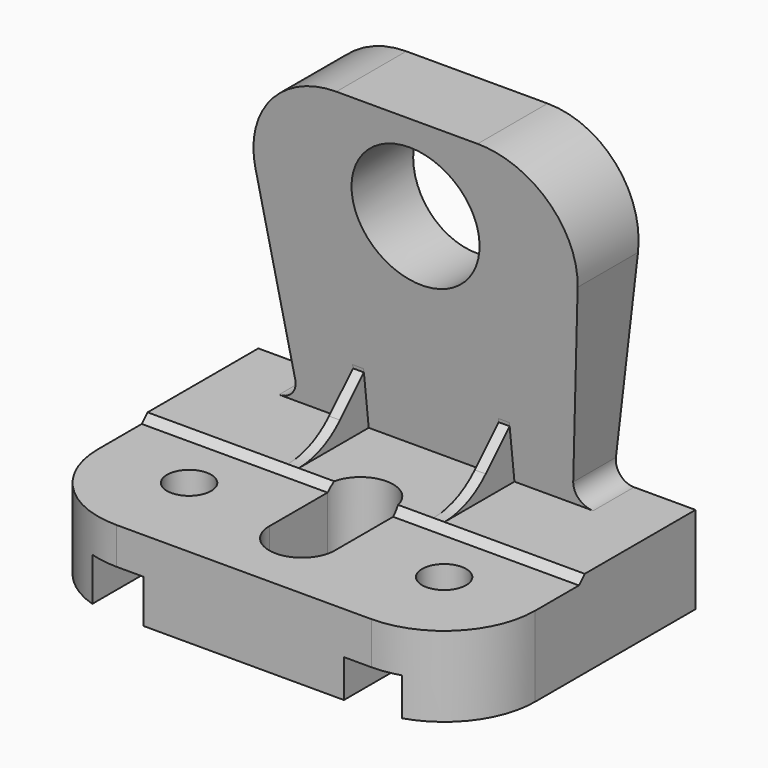
from build123d import *

# Parameters (mm, degrees)
F1_DEPTH      = 60
F2_W          = 15
F2_H          = 11.9018135592
F2_H_2        = 10.3764180094
F3_DEPTH      = 80.001
F5_DEPTH      = 80.001
F6_W          = 3
F6_H          = 15
F7_DEPTH      = 40
F9_DEPTH      = 60.001
F9_DEPTH_BACK = 60.001
F11_D         = 12.1
F13_DEPTH     = 109.001
F15_D         = 35
F16_R         = 25
F17_SIZE      = 1.99999


# Not quite as in the source:
# - a fillet or chamfer is up to 0.001 mm smaller than in the source, because OpenCascade refuses the exact size


with BuildPart() as f1:
    # F0 (on Right) → F1 (new body, symmetric)
    with BuildSketch(Plane.YZ):
        Polygon((-80, 0), (0, 0), (0, 109), (-24, 109), (-14.0000553612, 24), (-40, 24), (-40, 22), (-80, 22), align=None)
    extrude(amount=F1_DEPTH, both=True)

    # F2 (on Front) → F3 (cut, through all)
    with BuildSketch(Plane.XZ):
        with Locations((-35, 5.9509067796)):
            Rectangle(F2_W, F2_H)
        with Locations((35, 5.1882090047)):
            Rectangle(F2_W, F2_H_2)
    extrude(amount=F3_DEPTH, mode=Mode.SUBTRACT)

    # F4 (on Front) → F5 (cut, through all)
    with BuildSketch(Plane.XZ):
        with BuildLine():
            ThreePointArc((-43.1227148243, 24), (-39.3863385559, 25.6774268435), (-38.1569614274, 29.5842030478))
            Line((-38.1569614274, 29.5842030478), (-44.2151375018, 81.0789847612))
            ThreePointArc((-44.2151375018, 81.0789847612), (-38.0682518594, 100.6128657827), (-19.3863705172, 109))
            Line((-19.3863705172, 109), (0, 109))
            Line((0, 109), (19.3863705172, 109))
            ThreePointArc((19.3863705172, 109), (38.0682518594, 100.6128657827), (44.2151375018, 81.0789847612))
            Line((44.2151375018, 81.0789847612), (38.1569614274, 29.5842030478))
            ThreePointArc((38.1569614274, 29.5842030478), (39.3863385559, 25.6774268435), (43.1227148243, 24))
            Line((43.1227148243, 24), (60, 24))
            Line((60, 24), (60, 136.873498559))
            Line((60, 136.873498559), (-60, 136.873498559))
            Line((-60, 136.873498559), (-60, 24))
            Line((-60, 24), (-43.1227148243, 24))
        make_face()
    extrude(amount=F5_DEPTH, mode=Mode.SUBTRACT)

    # F6 (on Front) → F7 (join, through all)
    with BuildSketch(Plane.XZ):
        with Locations((-20, 31.5)):
            Rectangle(F6_W, F6_H)
        with Locations((20, 31.5)):
            Rectangle(F6_W, F6_H)
    extrude(amount=F7_DEPTH)

    # F8 (on Right) → F9 (cut, two sides)
    with BuildSketch(Plane.YZ) as f9_sk:
        with BuildLine():
            Line((-23.8578643763, 29.8578643763), (-15.6543285765, 38.061400176))
            Line((-15.6543285765, 38.061400176), (-16.3282091593, 43.7894168409))
            Line((-16.3282091593, 43.7894168409), (-43.991163373, 43.7894168409))
            Line((-43.991163373, 43.7894168409), (-43.991163373, 24))
            Line((-43.991163373, 24), (-38, 24))
            ThreePointArc((-38, 24), (-30.3463313527, 25.5224093498), (-23.8578643763, 29.8578643763))
        make_face()
    extrude(amount=-F9_DEPTH, mode=Mode.SUBTRACT)
    extrude(f9_sk.sketch, amount=F9_DEPTH_BACK, mode=Mode.SUBTRACT)

    # F11 (through all)
    with Locations(Plane(origin=(0, 0, 0), x_dir=(1, 0, 0), z_dir=(0, 0, -1))):
        with Locations((-35, 55), (35, 55)):
            Hole(F11_D / 2)

    # F12 (on Top) → F13 (cut, through all)
    with BuildSketch(Plane.XY):
        with BuildLine():
            Line((-9, -40), (-9, -60))
            ThreePointArc((-9, -60), (0, -69), (9, -60))
            Line((9, -60), (9, -40))
            ThreePointArc((9, -40), (0, -31), (-9, -40))
        make_face()
    extrude(amount=F13_DEPTH, mode=Mode.SUBTRACT)

    # F15 (through all)
    with Locations(Plane(origin=(0, 0, 0), x_dir=(1, 0, 0), z_dir=(0, 1, 0))):
        with Locations((0, -84)):
            Hole(F15_D / 2)

    # F16
    f16_edges = [f1.edges().sort_by_distance(p)[0] for p in [
        (-60, -80, 11),
        (60, -80, 11),
    ]]
    fillet(f16_edges, radius=F16_R)

    # F17 (size 2 in the source; OpenCascade refuses exactly that, so slightly less here)
    f17_edges = [f1.edges().sort_by_distance(p)[0] for p in [
        (34.5, -40, 24),
        (-34.5, -40, 24),
    ]]
    chamfer(f17_edges, length=F17_SIZE)


solid = f1.part
